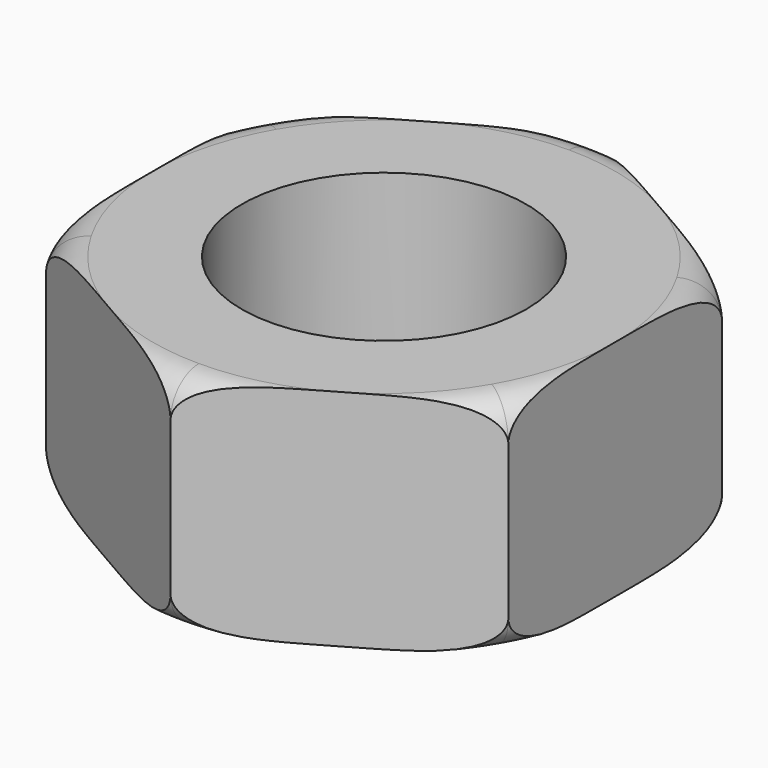
from build123d import *

# Parameters (mm, degrees)
F0_R     = 4
F1_DEPTH = 3.15
F2_R     = 1
F3_DEPTH = 3.5


with BuildPart() as f1:
    # F0 (on Top) → F1 (new body, symmetric)
    with BuildSketch(Plane.XY):
        with BuildLine():
            ThreePointArc((-6.5, 3.752777), (-7.505553, 0), (-6.5, -3.752777))
            Line((-6.5, -3.752777), (-6.5, 3.752777))
        make_face()
        with BuildLine():
            ThreePointArc((0, 7.505553), (-3.752777, 6.5), (-6.5, 3.752777))
            Line((-6.5, 3.752777), (0, 7.505553))
        make_face()
        with BuildLine():
            ThreePointArc((6.5, 3.752777), (3.752777, 6.5), (0, 7.505553))
            Line((0, 7.505553), (6.5, 3.752777))
        make_face()
        Polygon((-6.5, 3.752777), (-6.5, -3.752777), (0, -7.505553), (6.5, -3.752777), (6.5, 3.752777), (0, 7.505553), align=None)
        Circle(F0_R, mode=Mode.SUBTRACT)
        with BuildLine():
            Line((0, -7.505553), (-6.5, -3.752777))
            ThreePointArc((-6.5, -3.752777), (-3.752777, -6.5), (0, -7.505553))
        make_face()
        with BuildLine():
            Line((6.5, 3.752777), (6.5, -3.752777))
            ThreePointArc((6.5, -3.752777), (7.249808, -1.94258), (7.505553, 0))
            ThreePointArc((7.505553, 0), (7.249808, 1.94258), (6.5, 3.752777))
        make_face()
        with BuildLine():
            Line((6.5, -3.752777), (0, -7.505553))
            ThreePointArc((0, -7.505553), (3.752777, -6.5), (6.5, -3.752777))
        make_face()
    extrude(amount=F1_DEPTH, both=True)

    # F2
    f2_edges = [f1.edges().sort_by_distance(p)[0] for p in [
        (0, 7.505553, -3.15),
        (0, 7.505553, 3.15),
    ]]
    fillet(f2_edges, radius=F2_R)

    # F0 (on Top) → F3 (cut, symmetric)
    with BuildSketch(Plane.XY):
        with BuildLine():
            ThreePointArc((-6.5, 3.752777), (-7.505553, 0), (-6.5, -3.752777))
            Line((-6.5, -3.752777), (-6.5, 3.752777))
        make_face()
        with BuildLine():
            ThreePointArc((0, 7.505553), (-3.752777, 6.5), (-6.5, 3.752777))
            Line((-6.5, 3.752777), (0, 7.505553))
        make_face()
        with BuildLine():
            ThreePointArc((6.5, 3.752777), (3.752777, 6.5), (0, 7.505553))
            Line((0, 7.505553), (6.5, 3.752777))
        make_face()
        with BuildLine():
            Line((6.5, 3.752777), (6.5, -3.752777))
            ThreePointArc((6.5, -3.752777), (7.249808, -1.94258), (7.505553, 0))
            ThreePointArc((7.505553, 0), (7.249808, 1.94258), (6.5, 3.752777))
        make_face()
        with BuildLine():
            Line((6.5, -3.752777), (0, -7.505553))
            ThreePointArc((0, -7.505553), (3.752777, -6.5), (6.5, -3.752777))
        make_face()
        with BuildLine():
            Line((0, -7.505553), (-6.5, -3.752777))
            ThreePointArc((-6.5, -3.752777), (-3.752777, -6.5), (0, -7.505553))
        make_face()
    extrude(amount=F3_DEPTH, both=True, mode=Mode.SUBTRACT)


solid = f1.part
